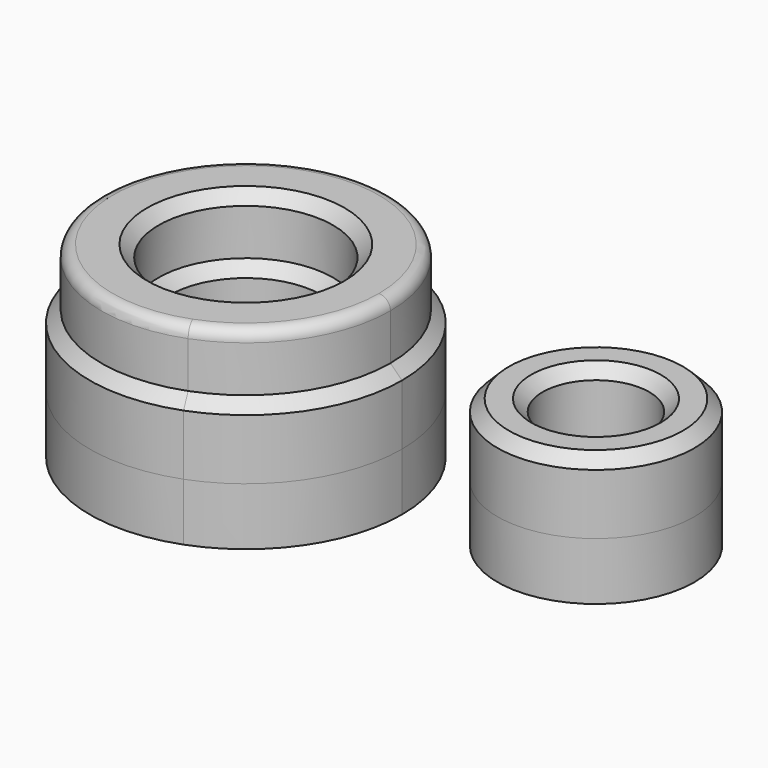
from build123d import *

# Parameters (mm, degrees)
F0_R      = 33.4031923569
F1_DEPTH  = 57.15
F0_R_2    = 23.5302271484
F2_DEPTH  = 25.4
F3_SIZE   = 5.08
F3_2_SIZE = 5.08
F4_DEPTH  = 25.4
F5_R      = 5.08
F6_SIZE   = 5.08


with BuildPart() as f1:
    # F0 (on Top) → F1 (new body)
    with BuildSketch(Plane.XY):
        with BuildLine():
            ThreePointArc((-111.4734922268, -88.070607267), (-79.0129136651, -62.8171326984), (-66.7329917311, -23.5662644833))
            ThreePointArc((-66.7329917311, -23.5662644833), (-85.9374640879, 24.1453452767), (-132.8404473474, 45.2479428834))
            ThreePointArc((-132.8404473474, 45.2479428834), (-203.6044087614, -34.4649077917), (-111.4734922268, -88.070607267))
        make_face()
        with Locations((-135.6026127041, -23.5662644833)):
            Circle(F0_R, mode=Mode.SUBTRACT)
    extrude(amount=F1_DEPTH)

    # F3
    f3_edges = [f1.edges().sort_by_distance(p)[0] for p in [
        (-159.731733, 40.938078, 0),
        (-111.473492, -88.070607, 28.575),
        (-159.731733, 40.938078, 57.15),
        (-169.005805, -23.566264, 57.15),
    ]]
    chamfer(f3_edges, length=F3_SIZE)

    # F4 (add): a face of the model
    f4_faces = [f1.faces().sort_by_distance(p)[0] for p in [
        (-157.3197738153, 34.4901908242, 57.15),
    ]]
    extrude(f4_faces, amount=F4_DEPTH)

    # F5
    f5_edges = [f1.edges().sort_by_distance(p)[0] for p in [
        (-157.951907, 36.180072, 82.55),
    ]]
    fillet(f5_edges, radius=F5_R)

    # F6
    f6_edges = [f1.edges().sort_by_distance(p)[0] for p in [
        (-174.085805, -23.566264, 82.55),
    ]]
    chamfer(f6_edges, length=F6_SIZE)


with BuildPart() as f1b:
    # F0 (on Top) → F1, piece 2 (new body)
    with BuildSketch(Plane.XY):
        with BuildLine():
            ThreePointArc((43.4512658516, 0), (-35.3357747424, 25.2862715216), (14.0207986405, -41.1269949011))
            ThreePointArc((14.0207986405, -41.1269949011), (35.3357747424, -25.2862715216), (43.4512658516, 0))
        make_face()
        Circle(F0_R_2, mode=Mode.SUBTRACT)
    extrude(amount=F1_DEPTH)

    # F3#2
    f3_2_edges = [f1b.edges().sort_by_distance(p)[0] for p in [
        (-14.020799, 41.126995, 57.15),
        (-23.530227, 0, 57.15),
    ]]
    chamfer(f3_2_edges, length=F3_2_SIZE)


with BuildPart() as f2:
    # F0 (on Top) → F2 (new body)
    with BuildSketch(Plane.XY):
        with BuildLine():
            ThreePointArc((-111.4734922268, -88.070607267), (-79.0129136651, -62.8171326984), (-66.7329917311, -23.5662644833))
            ThreePointArc((-66.7329917311, -23.5662644833), (-85.9374640879, 24.1453452767), (-132.8404473474, 45.2479428834))
            ThreePointArc((-132.8404473474, 45.2479428834), (-203.6044087614, -34.4649077917), (-111.4734922268, -88.070607267))
        make_face()
        with Locations((-135.6026127041, -23.5662644833)):
            Circle(F0_R, mode=Mode.SUBTRACT)
    extrude(amount=F2_DEPTH)


with BuildPart() as f2b:
    # F0 (on Top) → F2, piece 2 (new body)
    with BuildSketch(Plane.XY):
        with BuildLine():
            ThreePointArc((43.4512658516, 0), (-35.3357747424, 25.2862715216), (14.0207986405, -41.1269949011))
            ThreePointArc((14.0207986405, -41.1269949011), (35.3357747424, -25.2862715216), (43.4512658516, 0))
        make_face()
        Circle(F0_R_2, mode=Mode.SUBTRACT)
    extrude(amount=F2_DEPTH)


solid = Compound([f1.part, f1b.part, f2.part, f2b.part])
